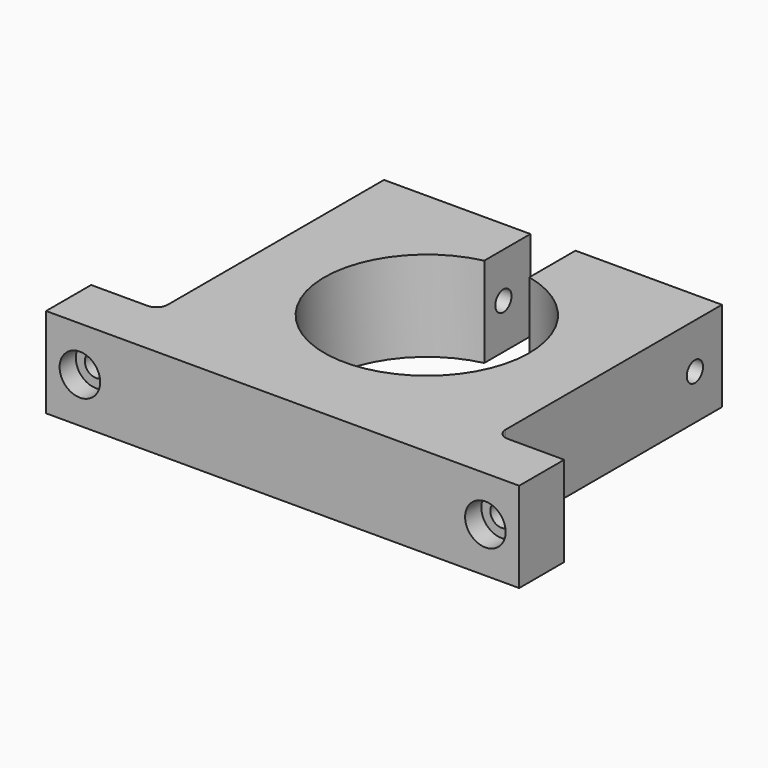
from build123d import *

# Parameters (mm, degrees)
F1_DEPTH  = 40
F2_R      = 45.5
F3_DEPTH  = 40.001
F4_W      = 20
F4_H      = 25.6125017601
F5_DEPTH  = 40.001
F6_R      = 4.5
F7_DEPTH  = 180.001
F8_R      = 5
F9_DEPTH  = 25.001
F10_R     = 9
F10_R_2   = 5
F11_DEPTH = 9
F12_R     = 5


# Not quite as in the source:
# - a pattern or mirror of a feature is missing from the dataset's text; its kind, count and spacing are read off the source's solid


with BuildPart() as f1:
    # F0 (on Top) → F1 (new body)
    with BuildSketch(Plane.XY):
        Polygon((-105, 25), (-105, 0), (105, 0), (105, 25), (75, 25), (75, 150), (-75, 150), (-75, 25), align=None)
    extrude(amount=F1_DEPTH)

    # F2 (on face) → F3 (cut, through all)
    with BuildSketch(Plane.XY.offset(40)):
        with Locations((0, 80)):
            Circle(F2_R)
    extrude(amount=-F3_DEPTH, mode=Mode.SUBTRACT)

    # F4 (on face) → F5 (cut, through all)
    with BuildSketch(Plane.XY.offset(40)):
        with Locations((0, 137.19374912)):
            Rectangle(F4_W, F4_H)
    extrude(amount=-F5_DEPTH, mode=Mode.SUBTRACT)

    # F6 (on face) → F7 (cut, through all)
    with BuildSketch(Plane.YZ.offset(75)):
        with Locations((135, 20)):
            Circle(F6_R)
    extrude(amount=-F7_DEPTH, mode=Mode.SUBTRACT)

    # F8 (on face) → F9 (cut, through all)
    with BuildSketch(Plane(origin=(0, 25, 0), x_dir=(-1, 0, 0), z_dir=(0, 1, 0))):
        with Locations((90, 20)):
            Circle(F8_R)
    f9 = extrude(amount=-F9_DEPTH, mode=Mode.SUBTRACT)

    # F9_copies: F9 across plane
    add(f9.mirror(Plane(origin=(0, 0, 0), x_dir=(0, 0, 1), z_dir=(1, 0, 0))), mode=Mode.SUBTRACT)

    # F10 (on face) → F11 (cut)
    with BuildSketch(Plane.XZ):
        with Locations((-90, 20)):
            Circle(F10_R)
        with Locations((-90, 20)):
            Circle(F10_R_2, mode=Mode.SUBTRACT)
    f11 = extrude(amount=-F11_DEPTH, mode=Mode.SUBTRACT)

    # F11_copies: F11 across plane
    add(f11.mirror(Plane(origin=(0, 0, 0), x_dir=(0, 0, 1), z_dir=(1, 0, 0))), mode=Mode.SUBTRACT)

    # F12
    f12_edges = [f1.edges().sort_by_distance(p)[0] for p in [
        (-75, 25, 20),
        (75, 25, 20),
    ]]
    fillet(f12_edges, radius=F12_R)


solid = f1.part
